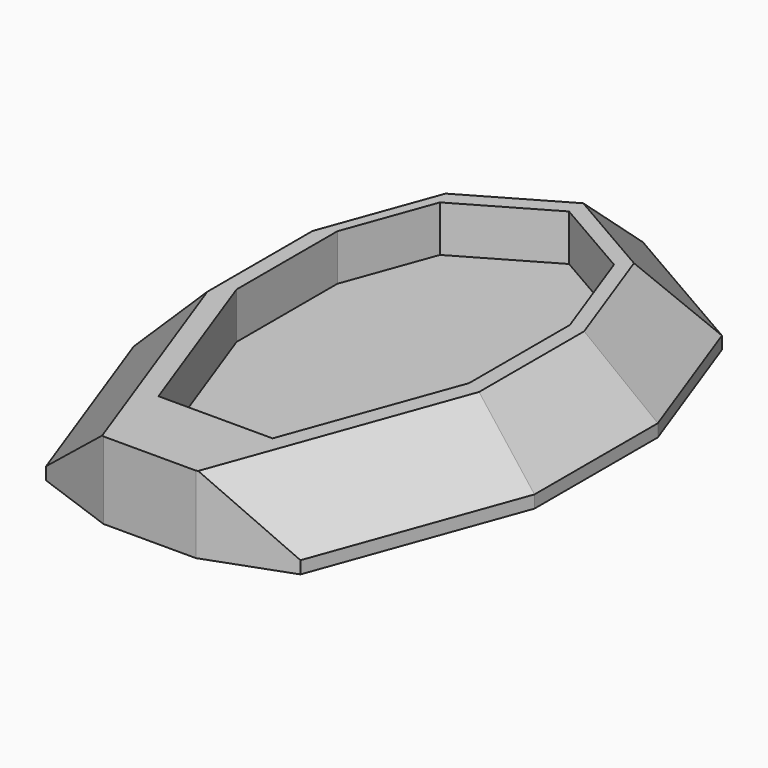
from build123d import *

# Parameters (mm, degrees)
F1_DEPTH = 10
F2_DEPTH = 90
F3_SIZE2 = 83.771
F3_SIZE  = 83.771
F5_DEPTH = 60


# Not quite as in the source:
# - a feature names something its author has since deleted; it is built from what else it names


with BuildPart() as f1:
    # F0 (on Top) → F1 (new body)
    with BuildSketch(Plane.XY):
        Polygon((190.5255888326, 290), (0, 400), (-190.5255888326, 290), (-260, 99.1206240876), (-260, -100.8793759124), (-165.0447262585, -361.7668463753), (-60, -400), (60, -400), (165.0447262585, -361.7668463753), (260, -100.8793759124), (260, 99.1206240876), align=None)
    extrude(amount=F1_DEPTH)

    # F2 (add): a face of the model
    f2_faces = [f1.faces().sort_by_distance(p)[0] for p in [
        (0, -14.4086757736, 10),
    ]]
    extrude(f2_faces, amount=F2_DEPTH)

    # F3
    f3_edges = [f1.edges().sort_by_distance(p)[0] for p in [
        (-212.522363, -231.323111, 100),
        (212.522363, -231.323111, 100),
        (260, -0.879376, 100),
        (225.262794, 194.560312, 100),
        (95.262794, 345, 100),
        (-95.262794, 345, 100),
        (-225.262794, 194.560312, 100),
        (-260, -0.879376, 100),
    ]]
    chamfer(f3_edges, length=F3_SIZE, length2=F3_SIZE2)

    # F4 (on face) → F5 (cut)
    with BuildSketch(Plane.XY.offset(100)):
        Polygon((-114.5740551886, 214.0262088265), (-156.229, 99.5801885487), (-156.229, -63.8245572211), (-71.6236926582, -296.2757287087), (76.4689935111, -296.2757287087), (156.229, -77.136911905), (156.229, 86.2678338648), (108.4396889686, 217.567886815), (0, 280.1755704318), align=None)
    extrude(amount=-F5_DEPTH, mode=Mode.SUBTRACT)


solid = f1.part
